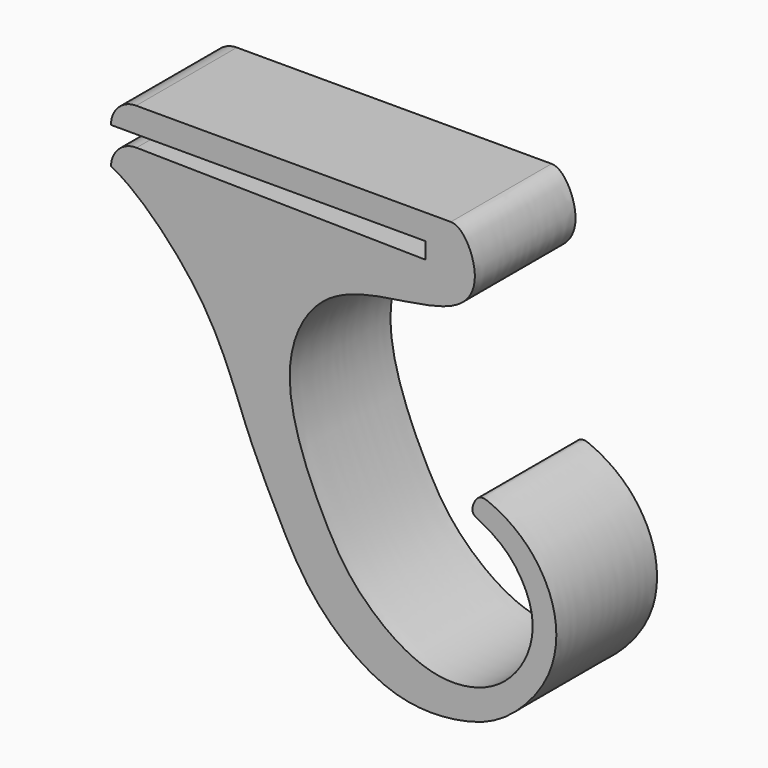
from build123d import *

# Parameters (mm, degrees)
F1_DEPTH    = 10
F2_T1_DEPTH = 20.0000328068
F2_T3_DEPTH = 20.1612799373


# Not quite as in the source:
# - a fillet or chamfer that OpenCascade refuses, or shapes differently, is made with other operations: its cross-section is extruded or revolved along the edge and cut away or added


with BuildPart() as f1:
    # F0 (on Front) → F1 (new body)
    with BuildSketch(Plane.XZ):
        with BuildLine():
            add(Edge.make_bspline(
                [(9.514e-06, -4.9000092057), (1.9342509703, -5.7788205185), (7.9600856629, -11.6080696819), (10.4938031921, -19.4137793601), (13.2500403785, -25.0265866718), (16.0500289635, -30.4023358123), (22.0167950969, -35.0563207405), (27.911105346, -34.8522886828), (31.7115032113, -33.387422259), (35.3435032228, -29.2143946597), (35.6055339141, -24.4460169523), (33.6592318937, -21.0363941268), (31.7383507436, -19.4689594446), (30.43406686, -18.7660216625), (29.3738509318, -18.3137291708), (28.816366228, -18.9329098548), (28.5876066373, -19.8493794371), (29.561159644, -20.2908633132), (31.9159451144, -21.6217051412), (34.4389998824, -26.1605857299), (31.5394611129, -31.68467843), (25.2994133189, -32.8268584607), (19.6574120082, -28.6533809644), (16.9014092861, -24.3354611486), (12.8798924189, -15.0223427162), (16.4183782289, -7.7481533751), (23.0483128553, -6.8018068739), (28.1506056372, -5.9724164167), (29.4354248767, -2.8544727466), (27.9299423215, -0.000363307), (27, 0)],
                knots=[0, 0, 0, 0, 0.05383222, 0.1044319916, 0.1467624797, 0.1890251708, 0.2352575736, 0.2757533164, 0.3100827924, 0.3493255944, 0.3860325166, 0.4195191391, 0.4462607539, 0.4672999815, 0.4844371334, 0.4989333801, 0.5141160934, 0.5300084197, 0.557950823, 0.5954379769, 0.6352941495, 0.6760815879, 0.7197508846, 0.7595802338, 0.813018719, 0.8582193053, 0.9017449186, 0.9396041953, 0.9688179628, 0.9999961563, 0.9999961563, 0.9999961563, 0.9999961563], degree=3))
            Line((27, 0), (27, -4.9000092057))
            Line((27, -4.9000092057), (9.514e-06, -4.9000092057))
        make_face()
        Polygon((26.9996560599, 0), (0, 0), (6.5614e-06, -2.0000092057), (25.0000065614, -2.0000092057), (25.0000065614, -3.3000092057), (9.514e-06, -2.9000092057), (9.514e-06, -4.9000092057), (27, -4.9000092057), (27, 0), align=None)
    extrude(amount=F1_DEPTH)

    # F2: fillet of radius 2 on 2 edges, made by hand

    # F2_s2 → F2_t1 (cut)
    with BuildSketch(Plane.XZ.offset(-5.0000164034)):
        with BuildLine():
            ThreePointArc((2.0000065614, 0), (0.5857906792, -0.5857887574), (6.5614e-06, -2.0000065613))
            Line((6.5614e-06, -2.0000065613), (0, 0))
            Line((0, 0), (2.0000065614, 0))
        make_face()
    extrude(amount=F2_T1_DEPTH, mode=Mode.SUBTRACT)

    # F2_s4 → F2_t3 (cut)
    with BuildSketch(Plane.XZ.offset(-5.0806399686)):
        with BuildLine():
            ThreePointArc((2.0320054225, -2.9325211441), (0.5971538224, -3.5067842537), (9.514e-06, -4.9322651931))
            Line((9.514e-06, -4.9322651931), (9.514e-06, -2.9000092057))
            Line((9.514e-06, -2.9000092057), (2.0320054225, -2.9325211441))
        make_face()
    extrude(amount=F2_T3_DEPTH, mode=Mode.SUBTRACT)


solid = f1.part
